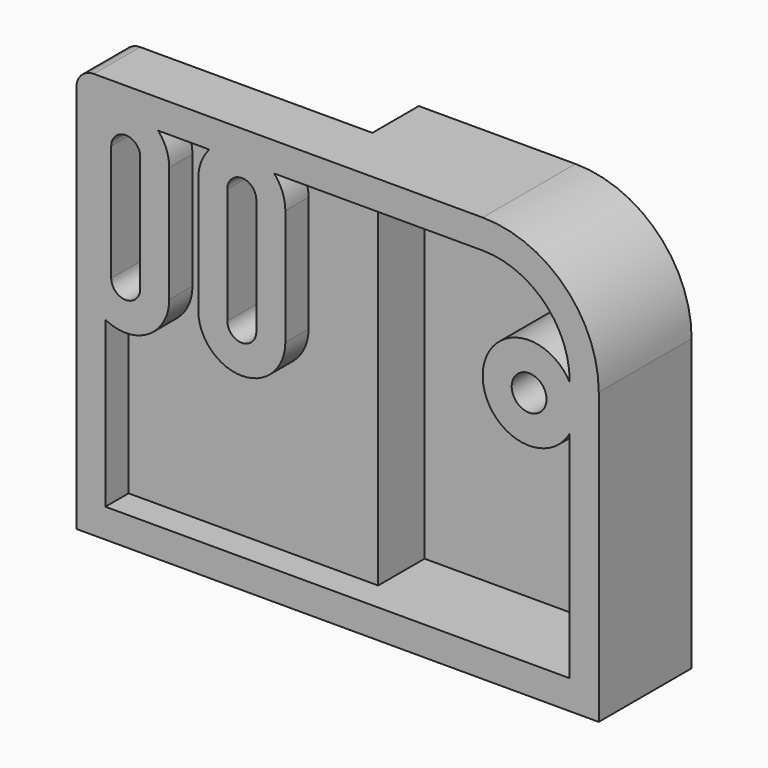
from build123d import *

# Parameters (mm, degrees)
F0_R        = 1.5
F1_DEPTH    = 10
F2_R        = 10
F0_W        = 21.5
F0_H        = 31.25
F3_DEPTH    = 5
F4_T        = 2.5
F4_T3_DEPTH = 26.5
F4_T5_DEPTH = 10
F4_T7_DEPTH = 36.25
F5_R        = 1.5


# Not quite as in the source:
# - a shell that OpenCascade refuses in one call is made with other operations: the cavity is built on its own and cut out


with BuildPart() as f1:
    # F0 (on Front) → F1 (new body)
    with BuildSketch(Plane.XZ):
        Polygon((25.1467653117, 20.7663856067), (1.6467653117, 20.7663856067), (1.6467653117, -10.4836143933), (-19.8532346883, -10.4836143933), (-19.8532346883, -14.2336143933), (25.1467653117, -14.2336143933), align=None)
        with Locations((19.1467653117, 8.7663856067)):
            Circle(F0_R, mode=Mode.SUBTRACT)
    extrude(amount=-F1_DEPTH)

    # F2
    f2_edges = [f1.edges().sort_by_distance(p)[0] for p in [
        (25.146765, 5, 20.766386),
    ]]
    fillet(f2_edges, radius=F2_R)

    # F0 (on Front) → F3 (join)
    with BuildSketch(Plane.XZ):
        with Locations((-9.1032346883, 5.1413856067)):
            Rectangle(F0_W, F0_H)
        with BuildLine():
            ThreePointArc((-16.8532346883, 15.7663856067), (-15.6032346883, 17.0163856067), (-14.3532346883, 15.7663856067))
            Line((-14.3532346883, 15.7663856067), (-14.3532346883, 5.7663856067))
            ThreePointArc((-14.3532346883, 5.7663856067), (-15.6032346883, 4.5163856067), (-16.8532346883, 5.7663856067))
            Line((-16.8532346883, 5.7663856067), (-16.8532346883, 15.7663856067))
        make_face(mode=Mode.SUBTRACT)
        with BuildLine():
            ThreePointArc((-6.8532346883, 15.7663856067), (-5.6032346883, 17.0163856067), (-4.3532346883, 15.7663856067))
            Line((-4.3532346883, 15.7663856067), (-4.3532346883, 5.7663856067))
            ThreePointArc((-4.3532346883, 5.7663856067), (-5.6032346883, 4.5163856067), (-6.8532346883, 5.7663856067))
            Line((-6.8532346883, 5.7663856067), (-6.8532346883, 15.7663856067))
        make_face(mode=Mode.SUBTRACT)
    extrude(amount=-F3_DEPTH)

    # F4: shell of thickness 2.5, made by hand


with BuildPart() as f4_core1:
    # F4_t2: copy of F1
    add(f1.part)

    # the walls: a layer under each face that stays
    f4_faces = [f4_core1.faces().sort_by_distance(p)[0] for p in [
        (25.1467653117, 5, -1.7336143933),
        (2.6467653117, 10, 3.2663856067),
        (17.6467653117, 5, 8.7663856067),
        (-9.1032346883, 7.5, -10.4836143933),
        (-9.1032346883, 5, 5.1413856067),
        (-5.6032346883, 2.5, 4.5163856067),
        (-4.3532346883, 2.5, 10.7663856067),
        (-5.6032346883, 2.5, 17.0163856067),
        (-6.8532346883, 2.5, 10.7663856067),
        (-15.6032346883, 2.5, 4.5163856067),
        (-14.3532346883, 2.5, 10.7663856067),
        (-15.6032346883, 2.5, 17.0163856067),
        (-16.8532346883, 2.5, 10.7663856067),
        (1.6467653117, 7.5, 5.1413856067),
        (-19.8532346883, 1.6666666667, 14.9330522734),
        (9.3134319783, 8.3333333333, 20.7663856067),
        (2.6467653117, 5, -14.2336143933),
        (22.2178331235, 5, 17.8374534186),
    ]]
    thicken(f4_faces, amount=-F4_T, mode=Mode.SUBTRACT)

    # F4_s4 → F4_t3 (cut)
    with BuildSketch(Plane.YZ.offset(-22.3532346883)):
        Polygon((5.025, -10.4586143933), (5, -12.9836143933), (2.5, -12.9836143933), (2.5, -10.4836143933), align=None)
    extrude(amount=F4_T3_DEPTH, mode=Mode.SUBTRACT)

    # F4_s6 → F4_t5 (cut)
    with BuildSketch(Plane.XZ.offset(-12.5)):
        Polygon((1.6217653117, -10.4586143933), (1.6467653117, -12.9836143933), (4.1467653117, -12.9836143933), (4.1467653117, -10.4836143933), align=None)
    extrude(amount=F4_T5_DEPTH, mode=Mode.SUBTRACT)

    # F4_s8 → F4_t7 (cut)
    with BuildSketch(Plane.XY.offset(-12.9836143933)):
        Polygon((1.6217653117, 5.025), (1.6467653117, 2.5), (4.1467653117, 2.5), (4.1467653117, 5), align=None)
    extrude(amount=F4_T7_DEPTH, mode=Mode.SUBTRACT)


with BuildPart() as f1_1:
    add(f1.part)

    # what is left inside the walls is the cavity
    f4_cavity = [f4_core1.part.solids().sort_by_distance(p)[0] for p in [
        (2.646765, 0.025, -1.733614),
    ]]
    add(f4_cavity, mode=Mode.SUBTRACT)

    # F5
    f5_edges = [f1_1.edges().sort_by_distance(p)[0] for p in [
        (-19.853235, 2.5, 20.766386),
    ]]
    fillet(f5_edges, radius=F5_R)


solid = f1_1.part
